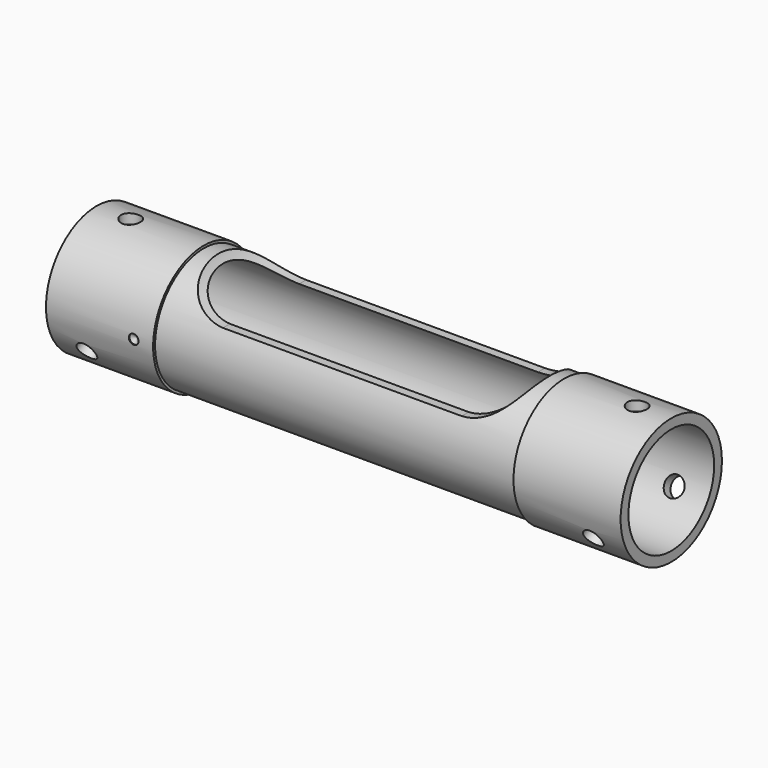
from build123d import *

# Parameters (mm, degrees)
F0_R      = 6.5
F0_R_2    = 5.5
F1_DEPTH  = 11
F2_R      = 6.25
F2_R_2    = 5.5
F3_DEPTH  = 37
F4_R      = 6.5
F4_R_2    = 6.25
F4_R_3    = 5.5
F5_DEPTH  = 11
F8_DEPTH  = 25
F10_D     = 1
F10_DEPTH = 0.1
F10_TIP   = 0.3004303095
F14_R     = 1
F15_DEPTH = 5
F17_R     = 1
F18_DEPTH = 5
F20_R     = 1
F21_DEPTH = 5
F25_R     = 1
F26_DEPTH = 5
F28_R     = 1
F29_DEPTH = 5
F31_R     = 1
F32_DEPTH = 5


with BuildPart() as f1:
    # F0 (on Right) → F1 (new body)
    with BuildSketch(Plane.YZ):
        Circle(F0_R)
        Circle(F0_R_2, mode=Mode.SUBTRACT)
    extrude(amount=F1_DEPTH)

    # F2 (on face) → F3 (join)
    with BuildSketch(Plane.YZ.offset(11)):
        Circle(F2_R)
        Circle(F2_R_2, mode=Mode.SUBTRACT)
    extrude(amount=F3_DEPTH)

    # F4 (on face) → F5 (join)
    with BuildSketch(Plane.YZ.offset(48)):
        Circle(F4_R)
        Circle(F4_R_2, mode=Mode.SUBTRACT)
        Circle(F4_R_2)
        Circle(F4_R_3, mode=Mode.SUBTRACT)
    extrude(amount=F5_DEPTH)

    # F7 (on offset) → F8 (cut)
    with BuildSketch(Plane.XZ.offset(6.5)):
        with BuildLine():
            Line((46.5, 6.25), (12.5, 6.25))
            ThreePointArc((12.5, 6.25), (14.469136254, 4.1135767851), (17.2433094418, 3.25))
            Line((17.2433094418, 3.25), (41.7566905582, 3.25))
            ThreePointArc((41.7566905582, 3.25), (44.530863746, 4.1135767851), (46.5, 6.25))
        make_face()
    extrude(amount=-F8_DEPTH, mode=Mode.SUBTRACT)

    # F10 (one way)
    with BuildSketch(Plane.XZ.offset(6.5)):
        with Locations((9, 0)):
            Circle(F10_D / 2)
    extrude(amount=-F10_DEPTH, mode=Mode.SUBTRACT)
    with Locations(Plane.XZ.offset(6.5)):
        with Locations((9, 0)):
            with Locations((0, 0, -(F10_DEPTH + F10_TIP / 2))):  # 118° drill point
                Cone(0, F10_D / 2, F10_TIP, mode=Mode.SUBTRACT)

    # F14 (on line) → F15 (cut)
    with BuildSketch(Plane.XY.offset(6.5)):
        with Locations((3.502298845, 0)):
            Circle(F14_R)
    extrude(amount=-F15_DEPTH, mode=Mode.SUBTRACT)

    # F17 (on line) → F18 (cut)
    with BuildSketch(Plane(origin=(0, 5.6291651246, -3.25), x_dir=(-1, 0, 0), z_dir=(0, 0.8660254038, -0.5))):
        with Locations((-3.5, 0)):
            Circle(F17_R)
    extrude(amount=-F18_DEPTH, mode=Mode.SUBTRACT)

    # F20 (on line) → F21 (cut)
    with BuildSketch(Plane(origin=(0, -5.6291651246, -3.25), x_dir=(1, 0, 0), z_dir=(0, -0.8660254038, -0.5))):
        with Locations((3.5, 0)):
            Circle(F20_R)
    extrude(amount=-F21_DEPTH, mode=Mode.SUBTRACT)

    # F25 (on line) → F26 (cut)
    with BuildSketch(Plane.XY.offset(6.5)):
        with Locations((55.5, 0)):
            Circle(F25_R)
    extrude(amount=-F26_DEPTH, mode=Mode.SUBTRACT)

    # F28 (on line) → F29 (cut)
    with BuildSketch(Plane(origin=(0, 5.6291651246, -3.25), x_dir=(-1, 0, 0), z_dir=(0, 0.8660254038, -0.5))):
        with Locations((-55.5, 0)):
            Circle(F28_R)
    extrude(amount=-F29_DEPTH, mode=Mode.SUBTRACT)

    # F31 (on line) → F32 (cut)
    with BuildSketch(Plane(origin=(0, -5.6291651246, -3.25), x_dir=(1, 0, 0), z_dir=(0, -0.8660254038, -0.5))):
        with Locations((55.5, 0)):
            Circle(F31_R)
    extrude(amount=-F32_DEPTH, mode=Mode.SUBTRACT)


solid = f1.part
